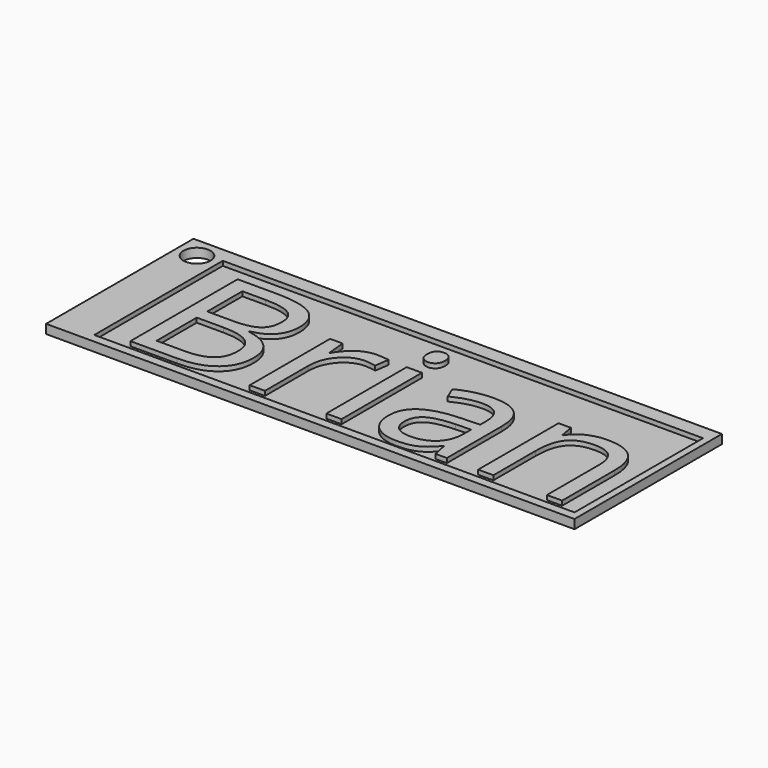
from build123d import *

# Parameters (mm, degrees)
F0_W         = 111.6905361414
F0_H         = 50.6127495319
F1_DEPTH     = 2
F2_R         = 3.0022801588
F3_DEPTH     = 25
F4_W         = 100.7550545037
F4_H         = 45.1337695122
F5_DEPTH     = 1
F7_DEPTH     = 5.5
F8_DEPTH     = 5.75
F6_TEXT_SIZE = 41.6171219614
F9_DEPTH     = 1
F10_DEPTH    = 9.5
F11_DEPTH    = 9.75


# Not quite as in the source:
# - Text() gives the source's letters only with a copy of the font that has no kerning and outlines rounded to 1/6400 em; it was checked with that copy


with BuildPart() as f1:
    # F0 (on Top) → F1 (new body)
    with BuildSketch(Plane.XY):
        with Locations((-0.6659552455, 4.8519736156)):
            Rectangle(F0_W, F0_H)
    extrude(amount=F1_DEPTH)

    # F2 (on face) → F3 (cut)
    with BuildSketch(Plane.XY.offset(2)):
        with Locations((-52.0630218089, 25.5633182824)):
            Circle(F2_R)
    extrude(amount=-F3_DEPTH, mode=Mode.SUBTRACT)

    # F4 (on face) → F5 (cut)
    with BuildSketch(Plane.XY.offset(2)):
        with Locations((2.9964316636, 4.3073724955)):
            Rectangle(F4_W, F4_H)
    extrude(amount=-F5_DEPTH, mode=Mode.SUBTRACT)

    # F7 (add): a face of the model
    f7_faces = [f1.faces().sort_by_distance(p)[0] for p in [
        (55.1793128252, 4.8519736156, 1),
    ]]
    extrude(f7_faces, amount=F7_DEPTH)

    # F8 (cut): a face of the model
    f8_faces = [f1.faces().sort_by_distance(p)[0] for p in [
        (53.3739589155, 4.3073724955, 1.5),
    ]]
    extrude(f8_faces, amount=-F8_DEPTH, mode=Mode.SUBTRACT)

    # F6 (on face) → F9 (join)
    with BuildSketch(Plane.XY.offset(1)):
        with Locations((-45.1337695122, -6.6483356059)):
            Text('Brian', F6_TEXT_SIZE, font='Open Sans', text_align=(TextAlign.LEFT, TextAlign.BOTTOM))
    extrude(amount=F9_DEPTH)

    # F10 (add): a face of the model
    f10_faces = [f1.faces().sort_by_distance(p)[0] for p in [
        (5.8714316636, -18.2595122606, 1.5),
    ]]
    extrude(f10_faces, amount=F10_DEPTH)

    # F11 (cut): a face of the model
    f11_faces = [f1.faces().sort_by_distance(p)[0] for p in [
        (2.0840447545, -20.4544011503, 1),
    ]]
    extrude(f11_faces, amount=-F11_DEPTH, mode=Mode.SUBTRACT)


solid = f1.part
